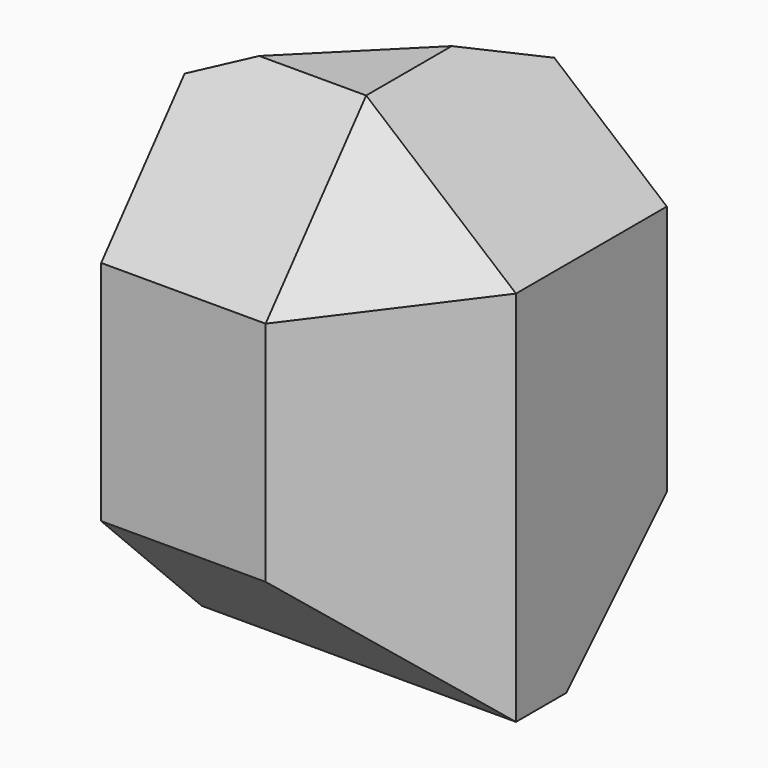
from build123d import *

# Parameters (mm, degrees)
F0_W        = 50
F0_H        = 50
F1_DEPTH    = 80
F2_T1_DEPTH = 27.2793198937
F2_T3_DEPTH = 202.8653193294
F2_T5_DEPTH = 172.8653193294
F2_T7_DEPTH = 172.8653193294
F3_SIZE     = 25
F4_SIZE     = 10
F5_SIZE     = 20


# Not quite as in the source:
# - a fillet or chamfer that OpenCascade refuses, or shapes differently, is made with other operations: its cross-section is extruded or revolved along the edge and cut away or added


with BuildPart() as f1:
    # F0 (on Top) → F1 (new body)
    with BuildSketch(Plane.XY):
        Rectangle(F0_W, F0_H)
    extrude(amount=F1_DEPTH)

    # F2: chamfer of 20 x 23.8350718519 on 3 edges, made by hand

    # F2_s2 → F2_t1 (cut)
    with BuildSketch(Plane(origin=(23.3481641649, -33.1608518108, 27.825258524), x_dir=(0.8176584321, 0.5757036463, 0), z_dir=(0.4747146788, -0.6742261621, 0.565742924))):
        Polygon((-13.4400778356, 34.368541497), (17.5629425707, 39.0194717243), (-1.9260049086, 63.2741944877), align=None)
    extrude(amount=F2_T1_DEPTH, mode=Mode.SUBTRACT)

    # F2_s4 → F2_t3 (cut)
    with BuildSketch(Plane.XY.offset(-61.4326596647)):
        Polygon((1.1649281481, -25), (25, -5), (25, -25), align=None)
    extrude(amount=F2_T3_DEPTH, mode=Mode.SUBTRACT)

    # F2_s6 → F2_t5 (cut)
    with BuildSketch(Plane.XZ.offset(-86.4326596647)):
        Polygon((25, 60), (1.1649281481, 80), (25, 80), align=None)
    extrude(amount=F2_T5_DEPTH, mode=Mode.SUBTRACT)

    # F2_s8 → F2_t7 (cut)
    with BuildSketch(Plane.YZ.offset(-86.4326596647)):
        Polygon((-25, 56.1649281481), (-5, 80), (-25, 80), align=None)
    extrude(amount=F2_T7_DEPTH, mode=Mode.SUBTRACT)

    # F3
    f3_edges = [f1.edges().sort_by_distance(p)[0] for p in [
        (-25, 25, 40),
    ]]
    chamfer(f3_edges, length=F3_SIZE)

    # F4
    f4_edges = [f1.edges().sort_by_distance(p)[0] for p in [
        (-12.5, 12.5, 80),
    ]]
    chamfer(f4_edges, length=F4_SIZE)

    # F5
    f5_edges = [f1.edges().sort_by_distance(p)[0] for p in [
        (12.5, 25, 0),
        (-11.917536, -25, 0),
    ]]
    chamfer(f5_edges, length=F5_SIZE)


solid = f1.part
